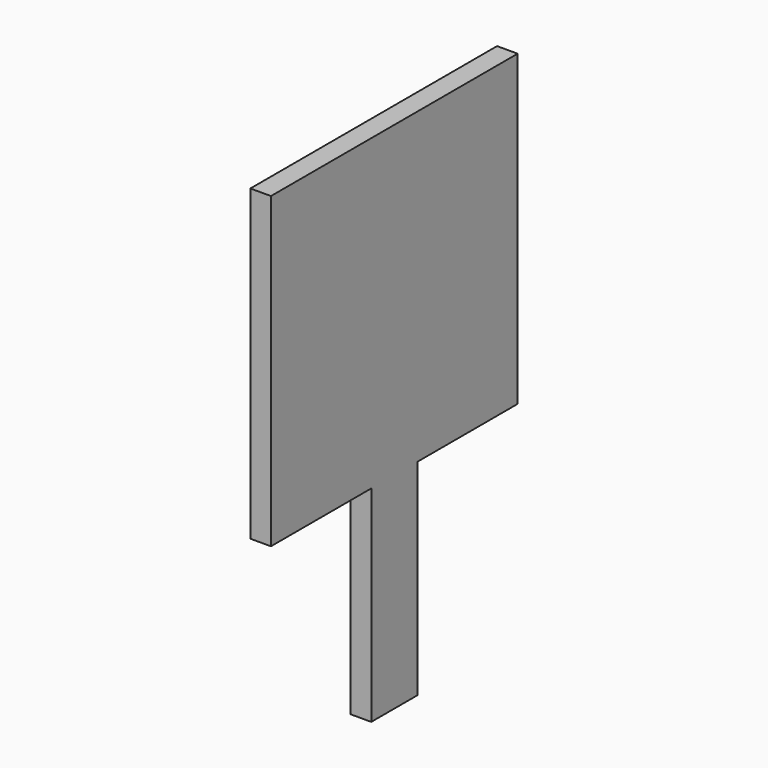
from build123d import *

# Parameters (mm, degrees)
F1_DEPTH = 1


# Not quite as in the source:
# - a feature names something its author has since deleted; it is built from what else it names


with BuildPart() as f1:
    # F0 (on Right) → F1 (new body)
    with BuildSketch(Plane.YZ):
        Polygon((11.5, 0), (0, 0), (-1.75, 0), (-1.75, -15), (0, -15), (4.35, -15), (4.35, -25), (5.25, -25), (6.25, -25), (7.15, -25), (7.15, -15), (11.5, -15), (13.25, -15), (13.25, 0), align=None)
    extrude(amount=F1_DEPTH)


solid = f1.part
